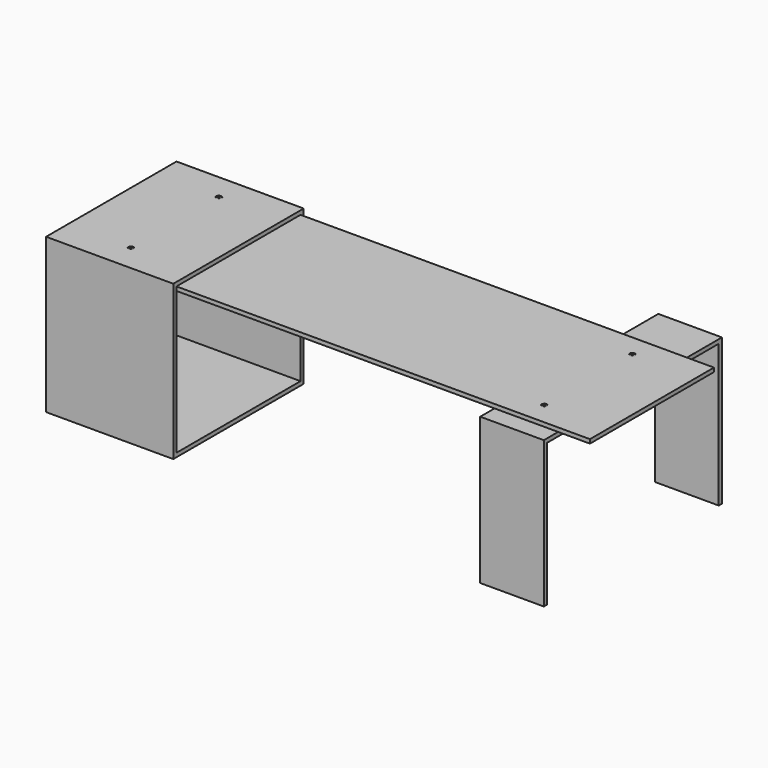
from build123d import *

# Parameters (mm, degrees)
F0_W          = 781.05
F0_H          = 739.775
F0_W_2        = 742.95
F0_H_2        = 701.675
F1_DEPTH      = 609.6
F2_W          = 742.95
F2_H          = 19.05
F3_DEPTH      = 2590.8
F4_W          = 304.8
F4_H          = 701.675
F5_DEPTH      = 457.2
F5_DEPTH_BACK = 609.6
F6_W          = 1028.7
F6_H          = 682.625
F7_DEPTH      = 2438.401
F8_R          = 12.7
F9_DEPTH      = 3.175
F10_R         = 12.7
F11_DEPTH     = 3.175
F12_R         = 3.175
F13_DEPTH     = 717.551
F14_R         = 3.175
F15_DEPTH     = 717.551
F16_R         = 3.175
F17_DEPTH     = 127
F19_R         = 3.175
F20_DEPTH     = 317.5


with BuildPart() as f1:
    # F0 (on Right) → F1 (new body)
    with BuildSketch(Plane.YZ):
        Rectangle(F0_W, F0_H)
        Rectangle(F0_W_2, F0_H_2, mode=Mode.SUBTRACT)
    extrude(amount=F1_DEPTH)

    # F8 (on face) → F9 (cut)
    with BuildSketch(Plane.XY.offset(369.8875)):
        with Locations((304.8, 263.525)):
            Circle(F8_R)
        with Locations((304.8, -263.525)):
            Circle(F8_R)
    extrude(amount=-F9_DEPTH, mode=Mode.SUBTRACT)


with BuildPart() as f3:
    # F2 (on Right) → F3 (new body)
    with BuildSketch(Plane.YZ):
        with Locations((0, 341.3125)):
            Rectangle(F2_W, F2_H)
    extrude(amount=F3_DEPTH)

    # F10 (on face) → F11 (cut)
    with BuildSketch(Plane.XY.offset(350.8375)):
        with Locations((2286, -263.525)):
            Circle(F10_R)
        with Locations((2286, 263.525)):
            Circle(F10_R)
    extrude(amount=-F11_DEPTH, mode=Mode.SUBTRACT)


with BuildPart() as f5:
    # F4 (on Front) → F5 (new body, two sides)
    with BuildSketch(Plane.XZ) as f5_sk:
        with Locations((2286, -19.05)):
            Rectangle(F4_W, F4_H)
    extrude(amount=F5_DEPTH)
    extrude(f5_sk.sketch, amount=-F5_DEPTH_BACK)

    # F6 (on face) → F7 (cut, through all)
    with BuildSketch(Plane.YZ.offset(2438.4)):
        with Locations((76.2, -28.575)):
            Rectangle(F6_W, F6_H)
    extrude(amount=-F7_DEPTH, mode=Mode.SUBTRACT)


with BuildPart() as f13_tool:
    # F12 (on face) → F13 (new body, through all)
    with BuildSketch(Plane.XY.offset(347.6625)):
        with Locations((2286, 263.525)):
            Circle(F12_R)
    extrude(amount=-F13_DEPTH)


with BuildPart() as f3_1:
    add(f3.part)

    # F13: cut by f13_tool
    add(f13_tool.part, mode=Mode.SUBTRACT)


with BuildPart() as f5_1:
    add(f5.part)

    # F13: cut by f13_tool
    add(f13_tool.part, mode=Mode.SUBTRACT)


with BuildPart() as f15_tool:
    # F14 (on face) → F15 (new body, through all)
    with BuildSketch(Plane.XY.offset(347.6625)):
        with Locations((2286, -263.525)):
            Circle(F14_R)
    extrude(amount=-F15_DEPTH)


with BuildPart() as f3_2:
    add(f3_1.part)

    # F15: cut by f15_tool
    add(f15_tool.part, mode=Mode.SUBTRACT)


with BuildPart() as f5_2:
    add(f5_1.part)

    # F15: cut by f15_tool
    add(f15_tool.part, mode=Mode.SUBTRACT)


with BuildPart() as f17_tool:
    # F16 (on face) → F17 (new body)
    with BuildSketch(Plane.XY.offset(366.7125)):
        with Locations((304.8, 263.525)):
            Circle(F16_R)
    extrude(amount=-F17_DEPTH)


with BuildPart() as f1_1:
    add(f1.part)

    # F17: cut by f17_tool
    add(f17_tool.part, mode=Mode.SUBTRACT)


with BuildPart() as f3_3:
    add(f3_2.part)

    # F17: cut by f17_tool
    add(f17_tool.part, mode=Mode.SUBTRACT)


with BuildPart() as f20_tool:
    # F19 (on face) → F20 (new body)
    with BuildSketch(Plane.XY.offset(366.7125)):
        with Locations((304.8, -263.525)):
            Circle(F19_R)
    extrude(amount=-F20_DEPTH)


with BuildPart() as f1_2:
    add(f1_1.part)

    # F20: cut by f20_tool
    add(f20_tool.part, mode=Mode.SUBTRACT)


with BuildPart() as f3_4:
    add(f3_3.part)

    # F20: cut by f20_tool
    add(f20_tool.part, mode=Mode.SUBTRACT)


solid = Compound([f5_2.part, f1_2.part, f3_4.part])
